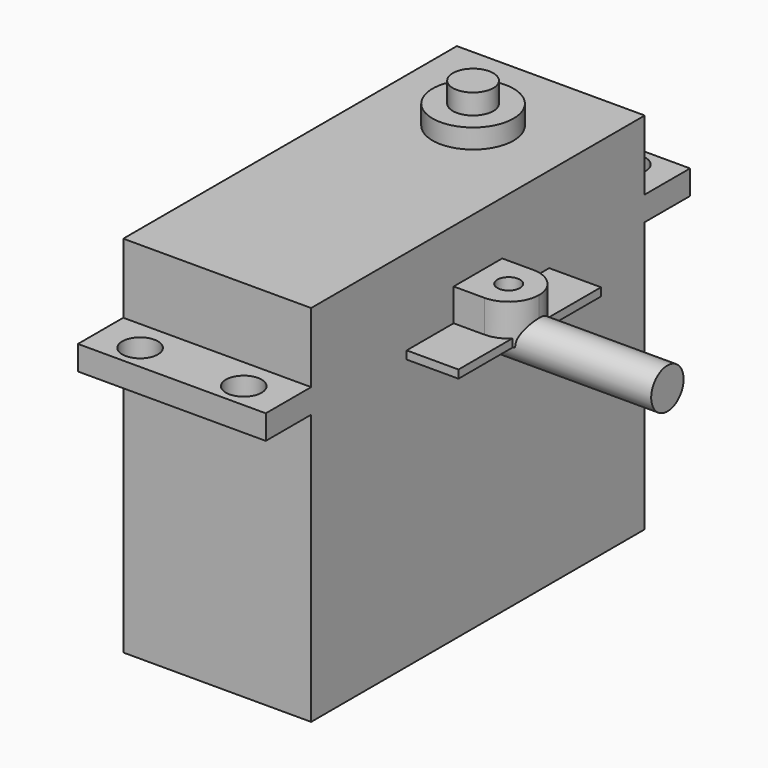
from build123d import *

# Parameters (mm, degrees)
F0_W      = 45.72
F0_H      = 27.94
F0_R      = 1.09
F1_DEPTH  = 1.27
F2_W      = 29.464
F2_H      = 8.89
F2_R      = 2.794
F2_H_2    = 65.405
F3_DEPTH  = 3.81
F4_DEPTH  = 14.732
F5_DEPTH  = 42.418
F6_R      = 3.175
F7_DEPTH  = 6.223
F6_R_2    = 6.35
F8_DEPTH  = 3.048
F9_W      = 6.35
F9_H      = 2.54
F10_DEPTH = 2.54
F11_R     = 3.175
F12_DEPTH = 44.45
F13_W     = 48.641
F13_H     = 9.525
F13_R     = 1.778
F14_DEPTH = 6.35
F15_R     = 4.76249


# Not quite as in the source:
# - a fillet or chamfer is up to 0.001 mm smaller than in the source, because OpenCascade refuses the exact size


with BuildPart() as f1:
    # F0 (on Top) → F1 (new body)
    with BuildSketch(Plane.XY):
        Rectangle(F0_W, F0_H)
        with Locations((19.86, -1.27)):
            Circle(F0_R, mode=Mode.SUBTRACT)
        with Locations((-20.68, 11.79)):
            Circle(F0_R, mode=Mode.SUBTRACT)
    extrude(amount=F1_DEPTH)


with BuildPart() as f3:
    # F2 (on Top) → F3 (new body)
    with BuildSketch(Plane.XY):
        with Locations((0, 37.1475)):
            Rectangle(F2_W, F2_H)
        with Locations((-8.128, 37.6555)):
            Circle(F2_R, mode=Mode.SUBTRACT)
        with Locations((8.128, 37.6555)):
            Circle(F2_R, mode=Mode.SUBTRACT)
        Rectangle(F2_W, F2_H_2)
        with Locations((0, -37.1475)):
            Rectangle(F2_W, F2_H)
        with Locations((-8.128, -37.6555)):
            Circle(F2_R, mode=Mode.SUBTRACT)
        with Locations((8.128, -37.6555)):
            Circle(F2_R, mode=Mode.SUBTRACT)
    extrude(amount=F3_DEPTH)

    # F2 (on Top) → F4 (join)
    with BuildSketch(Plane.XY):
        Rectangle(F2_W, F2_H_2)
    extrude(amount=F4_DEPTH)

    # F2 (on Top) → F5 (join)
    with BuildSketch(Plane.XY):
        Rectangle(F2_W, F2_H_2)
    extrude(amount=-F5_DEPTH)

    # F6 (on face) → F7 (join)
    with BuildSketch(Plane.XY.offset(14.732)):
        with Locations((0, 17.4625)):
            Circle(F6_R)
    extrude(amount=F7_DEPTH)

    # F6 (on face) → F8 (join)
    with BuildSketch(Plane.XY.offset(14.732)):
        with Locations((0, 17.4625)):
            Circle(F6_R_2)
        with Locations((0, 17.4625)):
            Circle(F6_R, mode=Mode.SUBTRACT)
    extrude(amount=F8_DEPTH)

    # F9 (on face) → F10 (join)
    with BuildSketch(Plane(origin=(0, 32.7025, 0), x_dir=(-1, 0, 0), z_dir=(0, 1, 0))):
        with Locations((0, -39.878)):
            Rectangle(F9_W, F9_H)
    extrude(amount=F10_DEPTH)


with BuildPart() as f12:
    # F11 (on Right) → F12 (new body)
    with BuildSketch(Plane.YZ):
        Circle(F11_R)
    extrude(amount=F12_DEPTH)


with BuildPart() as f14:
    # F13 (on Top) → F14 (new body)
    with BuildSketch(Plane.XY):
        Rectangle(F13_W, F13_H)
        with Locations((-19.558, 0)):
            Circle(F13_R, mode=Mode.SUBTRACT)
        with Locations((-9.779, 0)):
            Circle(F13_R, mode=Mode.SUBTRACT)
        Circle(F13_R, mode=Mode.SUBTRACT)
        with Locations((9.779, 0)):
            Circle(F13_R, mode=Mode.SUBTRACT)
        with Locations((19.558, 0)):
            Circle(F13_R, mode=Mode.SUBTRACT)
    extrude(amount=F14_DEPTH)

    # F15 (radius 4.7625 in the source; OpenCascade refuses exactly that, so slightly less here)
    f15_edges = [f14.edges().sort_by_distance(p)[0] for p in [
        (-24.3205, -4.7625, 3.175),
        (24.3205, -4.7625, 3.175),
        (24.3205, 4.7625, 3.175),
        (-24.3205, 4.7625, 3.175),
    ]]
    fillet(f15_edges, radius=F15_R)


solid = Compound([f1.part, f3.part, f12.part, f14.part])
